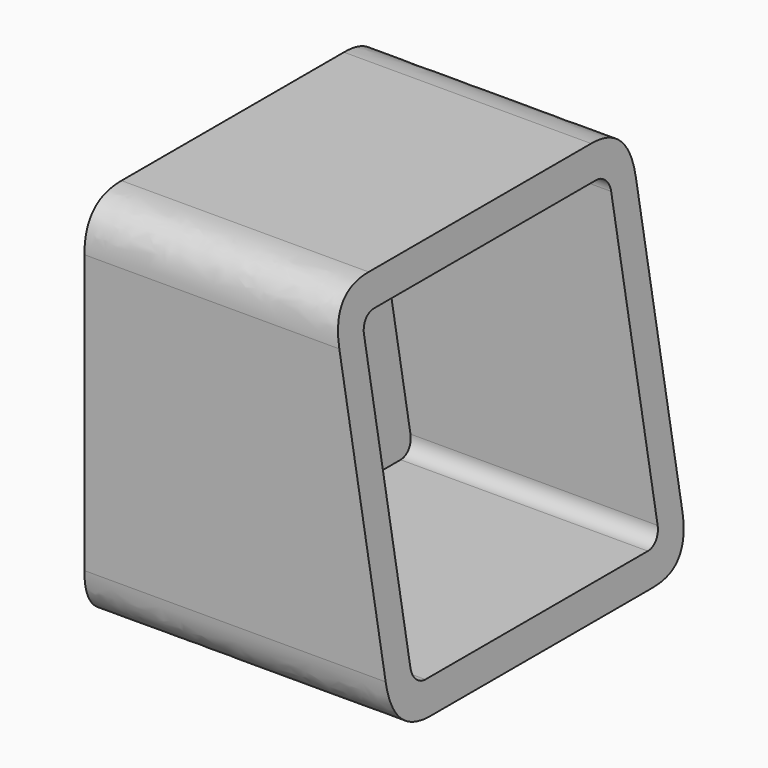
from build123d import *

# Parameters (mm, degrees)
F0_W        = 304.8
F0_H        = 304.8
F1_DEPTH    = 304.8
F3_DEPTH    = 304.801
F4_T1_DEPTH = 393.7
F4_T3_DEPTH = 444.5
F5_W        = 254
F5_H        = 258.2043365391
F7_R        = 12.7


# Not quite as in the source:
# - a fillet or chamfer that OpenCascade refuses, or shapes differently, is made with other operations: its cross-section is extruded or revolved along the edge and cut away or added


with BuildPart() as f1:
    # F0 (on Front) → F1 (new body)
    with BuildSketch(Plane.XZ):
        Rectangle(F0_W, F0_H)
    extrude(amount=F1_DEPTH)

    # F2 (on face) → F3 (cut, through all)
    with BuildSketch(Plane.XZ.offset(304.8)):
        Polygon((152.4, 152.4), (50.8, 152.4), (101.6, -152.4), (152.4, -152.4), align=None)
    extrude(amount=-F3_DEPTH, mode=Mode.SUBTRACT)

    # F4: fillet of radius 38.1 on 4 edges, made by hand

    # F4_s2 → F4_t1 (cut)
    with BuildSketch(Plane.YZ.offset(-247.65)):
        with BuildLine():
            add(Edge.make_bspline(
                [(-266.7, 152.4), (-304.8, 152.4), (-304.8, 114.3)],
                knots=[0, 0, 0, 1, 1, 1], degree=2, weights=[1, 1, 1]))
            Line((-304.8, 114.3), (-304.8, 152.4))
            Line((-304.8, 152.4), (-266.7, 152.4))
        make_face()
        with BuildLine():
            add(Edge.make_bspline(
                [(-38.1, 152.4), (0, 152.4), (0, 114.3)],
                knots=[0, 0, 0, 1, 1, 1], degree=2, weights=[1, 1, 1]))
            Line((0, 114.3), (0, 152.4))
            Line((0, 152.4), (-38.1, 152.4))
        make_face()
    extrude(amount=F4_T1_DEPTH, mode=Mode.SUBTRACT)

    # F4_s4 → F4_t3 (cut)
    with BuildSketch(Plane.YZ.offset(-247.65)):
        with BuildLine():
            add(Edge.make_bspline(
                [(0, -114.3), (0, -152.4), (-38.1, -152.4)],
                knots=[0, 0, 0, 1, 1, 1], degree=2, weights=[1, 1, 1]))
            Line((-38.1, -152.4), (0, -152.4))
            Line((0, -152.4), (0, -114.3))
        make_face()
        with BuildLine():
            add(Edge.make_bspline(
                [(-304.8, -114.3), (-304.8, -152.4), (-266.7, -152.4)],
                knots=[0, 0, 0, 1, 1, 1], degree=2, weights=[1, 1, 1]))
            Line((-266.7, -152.4), (-304.8, -152.4))
            Line((-304.8, -152.4), (-304.8, -114.3))
        make_face()
    extrude(amount=F4_T3_DEPTH, mode=Mode.SUBTRACT)

    # F6: sweep along a path in F6_path
    with BuildLine(Plane(origin=(50.8, -266.7, 152.4), x_dir=(0, -1, 0), z_dir=(0, 0, -1))) as f6_path:
        Line((0, 0), (0, 203.2))
    # F5 (on face) → F6 (sweep, cut)
    with BuildSketch(Plane(origin=(74.1405405405, 0, 12.3567567568), x_dir=(0, 1, 0), z_dir=(0.9863939238, 0, 0.1643989873))):
        with Locations((-152.4, -12.5272028327)):
            Rectangle(F5_W, F5_H)
    sweep(path=f6_path.line, mode=Mode.SUBTRACT)

    # F7
    f7_edges = [f1.edges().sort_by_distance(p)[0] for p in [
        (-4.175734, -279.4, -127.345594),
        (-4.175734, -25.4, -127.345594),
        (-46.624266, -279.4, 127.345594),
        (-46.624266, -25.4, 127.345594),
    ]]
    fillet(f7_edges, radius=F7_R)


solid = f1.part
